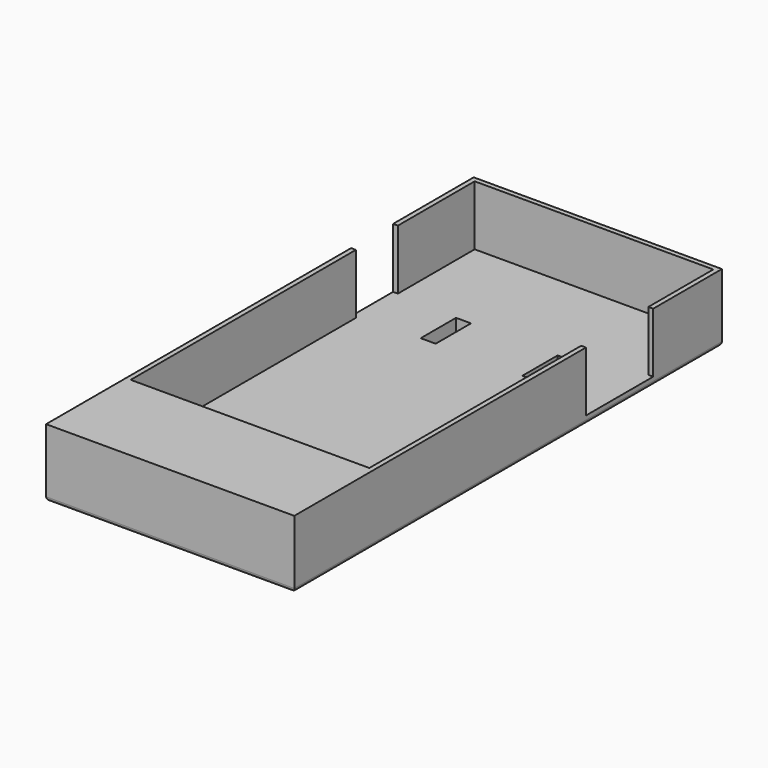
from build123d import *

# Parameters (mm, degrees)
F0_W     = 62.1875934303
F0_H     = 133.9231580496
F1_DEPTH = 2
F3_DEPTH = 15
F4_W     = 62.1875934303
F4_H     = 1.7857002169
F5_DEPTH = 25
F6_W     = 41.5440425277
F6_H     = 88.6942744255
F7_DEPTH = 2
F8_W     = 3.7540234625
F8_H     = 11.0563002527
F9_DEPTH = 8
F10_R    = 0.99999


# Not quite as in the source:
# - a fillet or chamfer is up to 0.001 mm smaller than in the source, because OpenCascade refuses the exact size


with BuildPart() as f1:
    # F0 (on Top) → F1 (new body)
    with BuildSketch(Plane.XY):
        Rectangle(F0_W, F0_H)
    extrude(amount=F1_DEPTH)

    # F2 (on face) → F3 (join)
    with BuildSketch(Plane.XY.offset(2)):
        Polygon((29.8937967151, 45.4372726381), (31.0937967151, 45.4372726381), (31.0937967151, 66.9615790248), (-31.0937967151, 66.9615790248), (-31.0937967151, 41.7135171592), (-29.8937967151, 41.7135171592), (-29.8937967151, 65.7615790248), (29.8937967151, 65.7615790248), align=None)
        Polygon((-31.0937967151, -66.9615790248), (31.0937967151, -66.9615790248), (31.0937967151, 24.3710856885), (29.8937967151, 24.3710856885), (29.8937967151, -65.7615790248), (-29.8937967151, -65.7615790248), (-29.8937967151, 28.5614430904), (-31.0937967151, 28.5614430904), align=None)
    extrude(amount=F3_DEPTH)

    # F4 (on face) → F5 (join)
    with BuildSketch(Plane.XZ.offset(66.9615790248)):
        with Locations((0, 16.1071498916)):
            Rectangle(F4_W, F4_H)
    extrude(amount=-F5_DEPTH)

    # F6 (on face) → F7 (join)
    with BuildSketch(Plane(origin=(0, 0, 0), x_dir=(1, 0, 0), z_dir=(0, 0, -1))):
        Rectangle(F6_W, F6_H)
    extrude(amount=F7_DEPTH)

    # F8 (on face) → F9 (cut)
    with BuildSketch(Plane(origin=(0, 0, -2), x_dir=(1, 0, 0), z_dir=(0, 0, -1))):
        with Locations((12.7368234098, -35.2913737297)):
            Rectangle(F8_W, F8_H)
        with Locations((-12.7368234098, -35.2913737297)):
            Rectangle(F8_W, F8_H)
        with Locations((-12.7368234098, 35.2913737297)):
            Rectangle(F8_W, F8_H)
        with Locations((12.7368234098, 35.2913737297)):
            Rectangle(F8_W, F8_H)
    extrude(amount=-F9_DEPTH, mode=Mode.SUBTRACT)

    # F10 (radius 1 in the source; OpenCascade refuses exactly that, so slightly less here)
    f10_edges = [f1.edges().sort_by_distance(p)[0] for p in [
        (0, -44.347137, -2),
        (20.772021, 0, -2),
        (-20.772021, 0, -2),
        (0, 44.347137, -2),
        (-10.859812, 35.291374, -2),
        (-12.736823, 29.763224, -2),
        (-14.613835, 35.291374, -2),
        (-12.736823, 40.819524, -2),
        (12.736823, 29.763224, -2),
        (10.859812, 35.291374, -2),
        (12.736823, 40.819524, -2),
        (14.613835, 35.291374, -2),
        (-12.736823, -29.763224, -2),
        (-10.859812, -35.291374, -2),
        (-12.736823, -40.819524, -2),
        (-14.613835, -35.291374, -2),
        (12.736823, -29.763224, -2),
        (14.613835, -35.291374, -2),
        (12.736823, -40.819524, -2),
        (10.859812, -35.291374, -2),
        (-31.093797, 0, 0),
        (0, 66.961579, 0),
        (0, -66.961579, 0),
        (31.093797, 0, 0),
        (20.772021, 0, 0),
        (0, 44.347137, 0),
        (-20.772021, 0, 0),
        (0, -44.347137, 0),
    ]]
    fillet(f10_edges, radius=F10_R)


solid = f1.part
